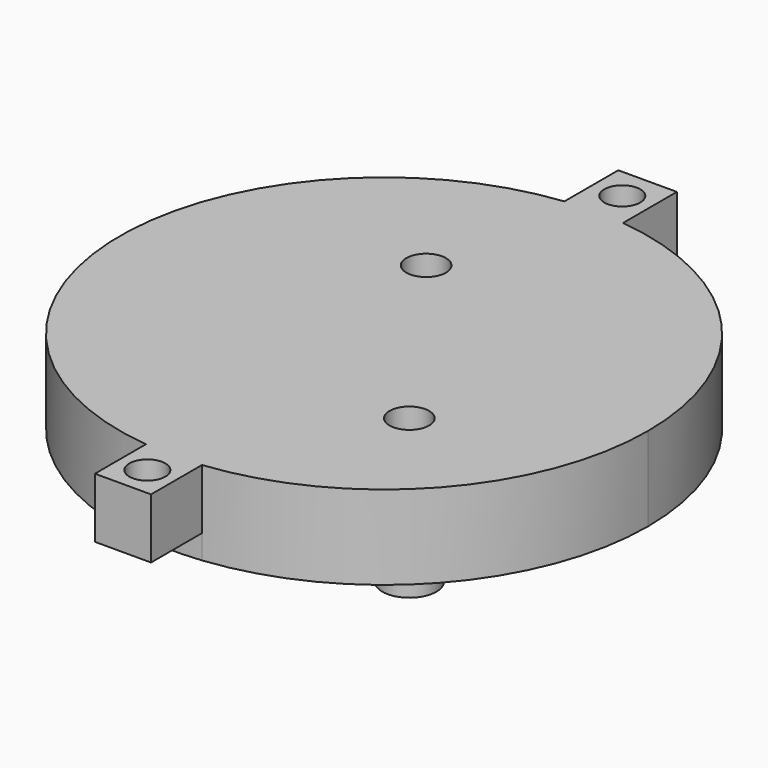
from build123d import *

# Parameters (mm, degrees)
F0_W     = 23.9
F0_H     = 23
F1_DEPTH = 7
F0_R     = 2.25
F2_DEPTH = 1
F3_W     = 12
F3_H     = 6
F4_DEPTH = 25
F5_R     = 21.25
F6_DEPTH = 10
F0_R_2   = 1.65
F7_DEPTH = 12
F0_R_3   = 1.5
F8_DEPTH = 5


# Not quite as in the source:
# - a feature names something its author has since deleted; it is built from what else it names


with BuildPart() as f1:
    # F0 (on Top) → F1 (new body)
    with BuildSketch(Plane.XY):
        with BuildLine():
            ThreePointArc((2.3312262639, -21.8761373214), (16.3598132295, -14.70906221), (22, 0))
            ThreePointArc((22, 0), (16.3897820024, 14.6756616857), (2.4204503716, 21.86644507))
            ThreePointArc((2.4204503716, 21.86644507), (-0.0200709954, 21.9999908444), (-2.4603446274, 21.8619922311))
            ThreePointArc((-2.4603446274, 21.8619922311), (-21.9999200002, -0.059329476), (-2.3423946746, -21.8749442785))
            ThreePointArc((-2.3423946746, -21.8749442785), (-0.0056159761, -21.9999992832), (2.3312262639, -21.8761373214))
        make_face()
        Rectangle(F0_W, F0_H, mode=Mode.SUBTRACT)
    extrude(amount=-F1_DEPTH)

    # F0 (on Top) → F2 (join)
    with BuildSketch(Plane.XY):
        Rectangle(F0_W, F0_H)
        with Locations((8.75, -8.3)):
            Circle(F0_R, mode=Mode.SUBTRACT)
        with Locations((-3.85, 9.2)):
            Circle(F0_R, mode=Mode.SUBTRACT)
    extrude(amount=-F2_DEPTH)

    # F3 (on face) → F4 (cut)
    with BuildSketch(Plane.YZ.offset(-11.95)):
        with Locations((0, -4.8)):
            Rectangle(F3_W, F3_H)
    extrude(amount=-F4_DEPTH, mode=Mode.SUBTRACT)

    # F5 (on face) → F6 (cut)
    with BuildSketch(Plane(origin=(0, 0, -1), x_dir=(1, 0, 0), z_dir=(0, 0, -1))):
        Circle(F5_R)
    extrude(amount=F6_DEPTH, mode=Mode.SUBTRACT)

    # F0 (on Top) → F7 (join)
    with BuildSketch(Plane.XY):
        with Locations((-3.85, 9.2)):
            Circle(F0_R)
        with Locations((-3.85, 9.2)):
            Circle(F0_R_2, mode=Mode.SUBTRACT)
        with Locations((8.75, -8.3)):
            Circle(F0_R)
        with Locations((8.75, -8.3)):
            Circle(F0_R_2, mode=Mode.SUBTRACT)
    extrude(amount=-F7_DEPTH)

    # F0 (on Top) → F8 (join)
    with BuildSketch(Plane.XY):
        with BuildLine():
            ThreePointArc((-2.4603446274, 21.8619922311), (-0.0200709954, 21.9999908444), (2.4204503716, 21.86644507))
            Line((2.4204503716, 21.86644507), (2.4204503716, 27.4773144078))
            Line((2.4204503716, 27.4773144078), (-2.4603446274, 27.4773144078))
            Line((-2.4603446274, 27.4773144078), (-2.4603446274, 21.8619922311))
        make_face()
        with Locations((0, 24.8148497194)):
            Circle(F0_R_3, mode=Mode.SUBTRACT)
        with BuildLine():
            Line((2.3312262639, -27.183307051), (2.3312262639, -21.8761373214))
            ThreePointArc((2.3312262639, -21.8761373214), (-0.0056159761, -21.9999992832), (-2.3423946746, -21.8749442785))
            Line((-2.3423946746, -21.8749442785), (-2.3423946746, -27.183307051))
            Line((-2.3423946746, -27.183307051), (2.3312262639, -27.183307051))
        make_face()
        with Locations((0, -24.6492363513)):
            Circle(F0_R_3, mode=Mode.SUBTRACT)
    extrude(amount=-F8_DEPTH)


solid = f1.part
